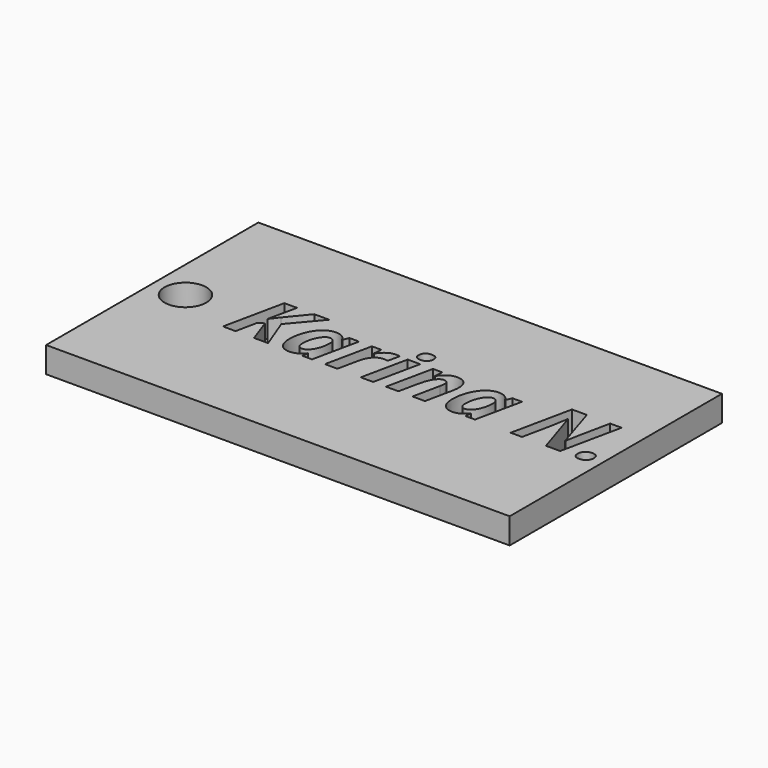
from build123d import *

# Parameters (mm, degrees)
F0_W         = 91.5222354233
F0_H         = 52.3806475103
F1_DEPTH     = 5.08
F2_R         = 4.1264929836
F2_TEXT_SIZE = 16.7886694221
F3_DEPTH     = 25.4


# Not quite as in the source:
# - Text() gives the source's letters only with a copy of the font that has no kerning and outlines rounded to 1/6400 em; it was checked with that copy


with BuildPart() as f1:
    # F0 (on Top) → F1 (new body)
    with BuildSketch(Plane.XY):
        with Locations((16.98054187, -0.2878047526)):
            Rectangle(F0_W, F0_H)
    extrude(amount=F1_DEPTH)

    # F2 (on face) → F3 (cut)
    with BuildSketch(Plane.XY.offset(5.08)):
        with Locations((-22.448848933, 0)):
            Circle(F2_R)
        with Locations((-11.8000358343, -4.6048923396)):
            Text('Karina N.', F2_TEXT_SIZE, font='Open Sans', font_style=FontStyle.BOLDITALIC, text_align=(TextAlign.LEFT, TextAlign.BOTTOM))
    extrude(amount=-F3_DEPTH, mode=Mode.SUBTRACT)


solid = f1.part
